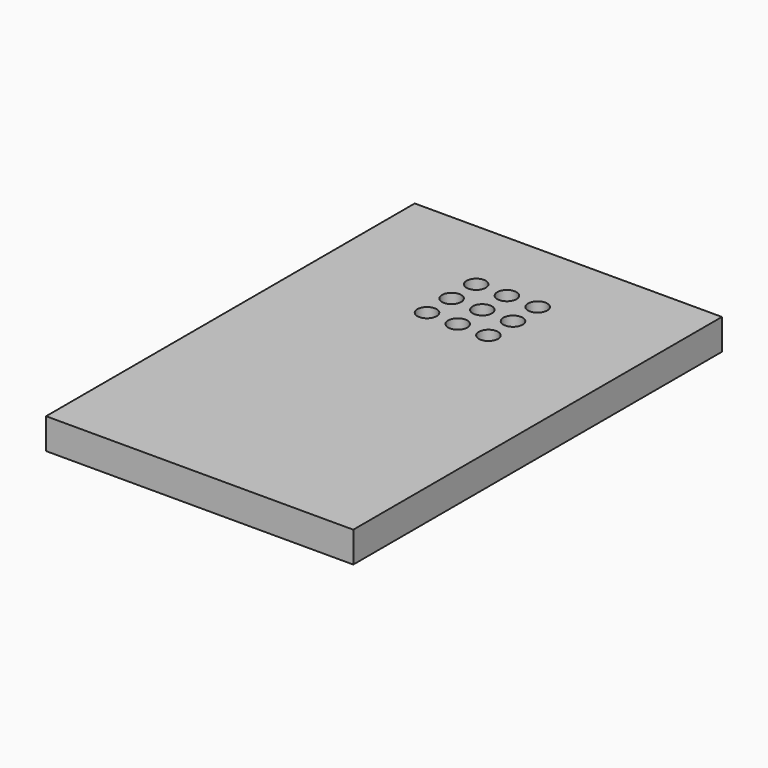
from build123d import *

# Parameters (mm, degrees)
F0_W     = 50.8
F0_H     = 76.2
F1_DEPTH = 5.08
F2_R     = 1.5875
F3_DEPTH = 76.2


# Not quite as in the source:
# - a feature names something its author has since deleted; it is built from what else it names


with BuildPart() as f1:
    # F0 (on Top) → F1 (new body)
    with BuildSketch(Plane.XY):
        with Locations((-14.0042318553, -16.4256663384)):
            Rectangle(F0_W, F0_H)
    extrude(amount=F1_DEPTH)

    # F2 (on face) → F3 (cut)
    with BuildSketch(Plane.XY.offset(5.08)):
        with Locations((-19.0842318553, 8.9743336616)):
            Circle(F2_R)
        with Locations((-14.0042318553, 8.9743336616)):
            Circle(F2_R)
        with Locations((-8.9242318553, 8.9743336616)):
            Circle(F2_R)
        with Locations((-19.0842318553, 3.8943336616)):
            Circle(F2_R)
        with Locations((-14.0042318553, 3.8943336616)):
            Circle(F2_R)
        with Locations((-8.9242318553, 3.8943336616)):
            Circle(F2_R)
        with Locations((-19.0842318553, -1.1856663384)):
            Circle(F2_R)
        with Locations((-14.0042318553, -1.1856663384)):
            Circle(F2_R)
        with Locations((-8.9242318553, -1.1856663384)):
            Circle(F2_R)
    extrude(amount=-F3_DEPTH, mode=Mode.SUBTRACT)


solid = f1.part
